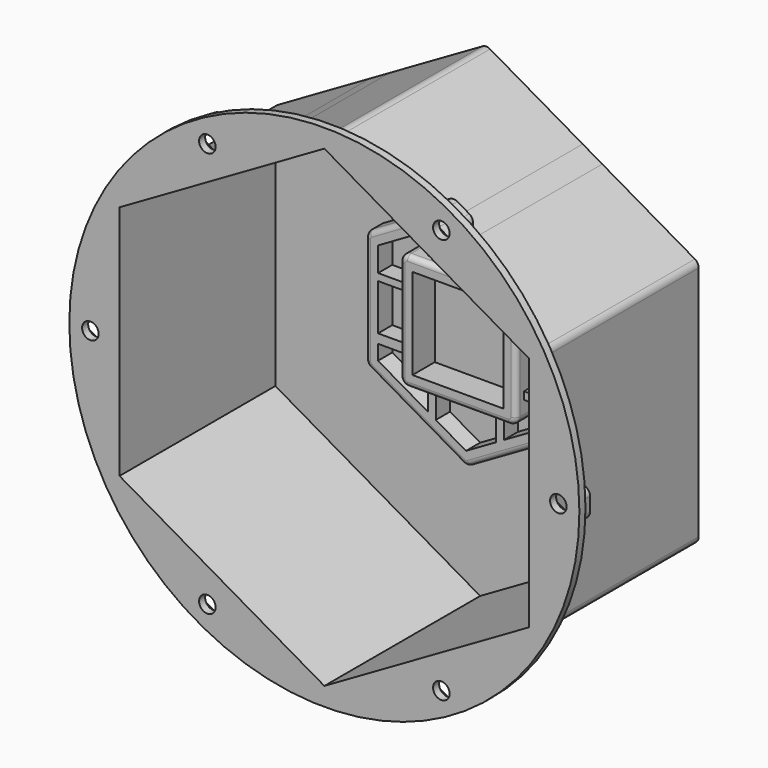
from build123d import *

# Parameters (mm, degrees)
F0_W      = 11.764
F0_H      = 3
F0_H_2    = 23.8
F0_H_3    = 3.6298790947
F0_H_4    = 18.1494033895
F0_H_5    = 2.7701719664
F1_DEPTH  = 3
F0_W_2    = 35.8
F0_H_6    = 35.8
F2_DEPTH  = 10
F3_DEPTH  = 79.8
F4_START  = 76.8
F0_R      = 100.55
F4_DEPTH  = 3
F5_R      = 2
F6_START  = 73.8
F0_W_3    = 0.8
F0_H_7    = 8.8911941455
F6_DEPTH  = 6
F7_D      = 6.5278
F8_DEPTH  = 14
F9_R      = 2
F10_DEPTH = 10


with BuildPart() as f1:
    # F0 (on Front) → F1 (new body)
    with BuildSketch(Plane.XZ):
        Polygon((0, -93.2420684741), (80.75, -46.6210342371), (80.75, 46.6210342371), (0, 93.2420684741), (-80.75, 46.6210342371), (-80.75, -46.6210342371), align=None)
        with BuildLine():
            ThreePointArc((39.664, -21.1679702696), (39.2620762114, -22.6679702696), (38.164, -23.7660464809))
            Line((38.164, -23.7660464809), (1.5, -44.9340167505))
            ThreePointArc((1.5, -44.9340167505), (0, -45.3359405391), (-1.5, -44.9340167505))
            Line((-1.5, -44.9340167505), (-38.164, -23.7660464809))
            ThreePointArc((-38.164, -23.7660464809), (-39.2620762114, -22.6679702696), (-39.664, -21.1679702696))
            Line((-39.664, -21.1679702696), (-39.664, 21.1679702696))
            ThreePointArc((-39.664, 21.1679702696), (-39.2620762114, 22.6679702696), (-38.164, 23.7660464809))
            Line((-38.164, 23.7660464809), (-1.5, 44.9340167505))
            ThreePointArc((-1.5, 44.9340167505), (0, 45.3359405391), (1.5, 44.9340167505))
            Line((1.5, 44.9340167505), (2.7712812921, 44.2000421543))
            Line((2.7712812921, 44.2000421543), (5.8889727457, 42.4000421543))
            Line((5.8889727457, 42.4000421543), (33.7750272543, 26.3000210771))
            Line((33.7750272543, 26.3000210771), (36.8927187079, 24.5000210771))
            Line((36.8927187079, 24.5000210771), (38.164, 23.7660464809))
            ThreePointArc((38.164, 23.7660464809), (39.2620762114, 22.6679702696), (39.664, 21.1679702696))
            Line((39.664, 21.1679702696), (39.664, -21.1679702696))
        make_face(mode=Mode.SUBTRACT)
        with BuildLine():
            Line((34.664, -20.0132697312), (34.664, -14.9))
            Line((34.664, -14.9), (22.9, -14.9))
            Line((22.9, -14.9), (22.9, -19.9))
            ThreePointArc((22.9, -19.9), (22.0213203436, -22.0213203436), (19.9, -22.9))
            Line((19.9, -22.9), (14.9, -22.9))
            Line((14.9, -22.9), (14.9, -31.4240204515))
            Line((14.9, -31.4240204515), (34.664, -20.0132697312))
        make_face()
        Polygon((11.9, -33.156071259), (14.9, -31.4240204515), (14.9, -22.9), (11.9, -22.9), align=None)
        Polygon((0, -40.0265394624), (11.9, -33.156071259), (11.9, -22.9), (-11.9, -22.9), (-11.9, -33.156071259), align=None)
        with BuildLine():
            Line((-14.9, 22.9), (-14.9, 31.4240204515))
            Line((-14.9, 31.4240204515), (-34.664, 20.0132697312))
            Line((-34.664, 20.0132697312), (-34.664, 10.4067251086))
            Line((-34.664, 10.4067251086), (-22.9, 10.4067251086))
            Line((-22.9, 10.4067251086), (-22.9, 19.9))
            ThreePointArc((-22.9, 19.9), (-22.0213203436, 22.0213203436), (-19.9, 22.9))
            Line((-19.9, 22.9), (-14.9, 22.9))
        make_face()
        Polygon((-11.9, 22.9), (-11.9, 33.156071259), (-14.9, 31.4240204515), (-14.9, 22.9), align=None)
        Polygon((11.9, 33.156071259), (3.3889727457, 38.0699151354), (0.2712812921, 39.8699151354), (0, 40.0265394624), (-11.9, 33.156071259), (-11.9, 22.9), (11.9, 22.9), align=None)
        Polygon((14.9, 22.9), (14.9, 31.4240204515), (11.9, 33.156071259), (11.9, 22.9), align=None)
        with BuildLine():
            Line((34.664, 20.0132697312), (34.3927187079, 20.1698940582))
            Line((34.3927187079, 20.1698940582), (31.2750272543, 21.9698940582))
            Line((31.2750272543, 21.9698940582), (14.9, 31.4240204515))
            Line((14.9, 31.4240204515), (14.9, 22.9))
            Line((14.9, 22.9), (19.9, 22.9))
            ThreePointArc((19.9, 22.9), (22.0213203436, 22.0213203436), (22.9, 19.9))
            Line((22.9, 19.9), (22.9, 14.9))
            Line((22.9, 14.9), (34.664, 14.9))
            Line((34.664, 14.9), (34.664, 20.0132697312))
        make_face()
        with Locations((28.782, 13.4)):
            Rectangle(F0_W, F0_H)
        with Locations((28.782, 0)):
            Rectangle(F0_W, F0_H_2)
        with Locations((28.782, -13.4)):
            Rectangle(F0_W, F0_H)
        Polygon((-14.9, -31.4240204515), (-11.9, -33.156071259), (-11.9, -22.9), (-14.9, -22.9), align=None)
        with BuildLine():
            Line((-22.9, -14.142729342), (-34.664, -14.142729342))
            Line((-34.664, -14.142729342), (-34.664, -20.0132697312))
            Line((-34.664, -20.0132697312), (-14.9, -31.4240204515))
            Line((-14.9, -31.4240204515), (-14.9, -22.9))
            Line((-14.9, -22.9), (-19.9, -22.9))
            ThreePointArc((-19.9, -22.9), (-22.0213203436, -22.0213203436), (-22.9, -19.9))
            Line((-22.9, -19.9), (-22.9, -14.142729342))
        make_face()
        with Locations((-28.782, -12.3277897947)):
            Rectangle(F0_W, F0_H_3)
        with Locations((-28.782, -1.4381485526)):
            Rectangle(F0_W, F0_H_4)
        with Locations((-28.782, 9.0216391254)):
            Rectangle(F0_W, F0_H_5)
        Polygon((3.3889727457, 38.0699151354), (5.8889727457, 42.4000421543), (2.7712812921, 44.2000421543), (0.2712812921, 39.8699151354), align=None)
        Polygon((34.3927187079, 20.1698940582), (36.8927187079, 24.5000210771), (33.7750272543, 26.3000210771), (31.2750272543, 21.9698940582), align=None)
    extrude(amount=F1_DEPTH)

    # F0 (on Front) → F2 (join)
    with BuildSketch(Plane.XZ):
        with BuildLine():
            Line((1.5, -44.9340167505), (38.164, -23.7660464809))
            ThreePointArc((38.164, -23.7660464809), (39.2620762114, -22.6679702696), (39.664, -21.1679702696))
            Line((39.664, -21.1679702696), (39.664, 21.1679702696))
            ThreePointArc((39.664, 21.1679702696), (39.2620762114, 22.6679702696), (38.164, 23.7660464809))
            Line((38.164, 23.7660464809), (36.8927187079, 24.5000210771))
            Line((36.8927187079, 24.5000210771), (34.3927187079, 20.1698940582))
            Line((34.3927187079, 20.1698940582), (34.664, 20.0132697312))
            Line((34.664, 20.0132697312), (34.664, 14.9))
            Line((34.664, 14.9), (34.664, 11.9))
            Line((34.664, 11.9), (34.664, -11.9))
            Line((34.664, -11.9), (34.664, -14.9))
            Line((34.664, -14.9), (34.664, -20.0132697312))
            Line((34.664, -20.0132697312), (14.9, -31.4240204515))
            Line((14.9, -31.4240204515), (11.9, -33.156071259))
            Line((11.9, -33.156071259), (0, -40.0265394624))
            Line((0, -40.0265394624), (-11.9, -33.156071259))
            Line((-11.9, -33.156071259), (-14.9, -31.4240204515))
            Line((-14.9, -31.4240204515), (-34.664, -20.0132697312))
            Line((-34.664, -20.0132697312), (-34.664, -14.142729342))
            Line((-34.664, -14.142729342), (-34.664, -10.5128502473))
            Line((-34.664, -10.5128502473), (-34.664, 7.6365531422))
            Line((-34.664, 7.6365531422), (-34.664, 10.4067251086))
            Line((-34.664, 10.4067251086), (-34.664, 20.0132697312))
            Line((-34.664, 20.0132697312), (-14.9, 31.4240204515))
            Line((-14.9, 31.4240204515), (-11.9, 33.156071259))
            Line((-11.9, 33.156071259), (0, 40.0265394624))
            Line((0, 40.0265394624), (0.2712812921, 39.8699151354))
            Line((0.2712812921, 39.8699151354), (2.7712812921, 44.2000421543))
            Line((2.7712812921, 44.2000421543), (1.5, 44.9340167505))
            ThreePointArc((1.5, 44.9340167505), (0, 45.3359405391), (-1.5, 44.9340167505))
            Line((-1.5, 44.9340167505), (-38.164, 23.7660464809))
            ThreePointArc((-38.164, 23.7660464809), (-39.2620762114, 22.6679702696), (-39.664, 21.1679702696))
            Line((-39.664, 21.1679702696), (-39.664, -21.1679702696))
            ThreePointArc((-39.664, -21.1679702696), (-39.2620762114, -22.6679702696), (-38.164, -23.7660464809))
            Line((-38.164, -23.7660464809), (-1.5, -44.9340167505))
            ThreePointArc((-1.5, -44.9340167505), (0, -45.3359405391), (1.5, -44.9340167505))
        make_face()
    extrude(amount=F2_DEPTH)

    # F0 (on Front) → F3 (join)
    with BuildSketch(Plane.XZ):
        with BuildLine():
            Line((83.75, 4.4455970728), (83.75, 46.6210342371))
            ThreePointArc((83.75, 46.6210342371), (83.3480762114, 48.1210342371), (82.25, 49.2191104484))
            Line((82.25, 49.2191104484), (45.725, 70.3068290306))
            Line((45.725, 70.3068290306), (38.025, 74.7524261033))
            Line((38.025, 74.7524261033), (1.5, 95.8401446855))
            ThreePointArc((1.5, 95.8401446855), (0, 96.2420684741), (-1.5, 95.8401446855))
            Line((-1.5, 95.8401446855), (-38.025, 74.7524261033))
            Line((-38.025, 74.7524261033), (-45.725, 70.3068290306))
            Line((-45.725, 70.3068290306), (-82.25, 49.2191104484))
            ThreePointArc((-82.25, 49.2191104484), (-83.3480762114, 48.1210342371), (-83.75, 46.6210342371))
            Line((-83.75, 46.6210342371), (-83.75, 4.1800841187))
            Line((-83.75, 4.1800841187), (-83.75, -3.9581455377))
            Line((-83.75, -3.9581455377), (-83.75, -46.6210342371))
            ThreePointArc((-83.75, -46.6210342371), (-83.3480762114, -48.1210342371), (-82.25, -49.2191104484))
            Line((-82.25, -49.2191104484), (-45.7833874392, -70.2731190268))
            Line((-45.7833874392, -70.2731190268), (-38.0831462279, -74.718855363))
            Line((-38.0831462279, -74.718855363), (-1.5, -95.8401446855))
            ThreePointArc((-1.5, -95.8401446855), (0, -96.2420684741), (1.5, -95.8401446855))
            Line((1.5, -95.8401446855), (38.1444882108, -74.6834395526))
            Line((38.1444882108, -74.6834395526), (45.8568599601, -70.2306996471))
            Line((45.8568599601, -70.2306996471), (82.25, -49.2191104484))
            ThreePointArc((82.25, -49.2191104484), (83.3480762114, -48.1210342371), (83.75, -46.6210342371))
            Line((83.75, -46.6210342371), (83.75, -4.4455970728))
            Line((83.75, -4.4455970728), (83.75, 4.4455970728))
        make_face()
        Polygon((80.75, 46.6210342371), (80.75, -46.6210342371), (0, -93.2420684741), (-80.75, -46.6210342371), (-80.75, 46.6210342371), (0, 93.2420684741), align=None, mode=Mode.SUBTRACT)
    extrude(amount=F3_DEPTH)

    # F0 (on Front) → F4 (join)
    with BuildSketch(Plane.XZ.offset(F4_START)):
        Circle(F0_R)
        with BuildLine():
            ThreePointArc((82.25, 49.2191104484), (83.3480762114, 48.1210342371), (83.75, 46.6210342371))
            Line((83.75, 46.6210342371), (83.75, 4.4455970728))
            Line((83.75, 4.4455970728), (84.55, 4.4455970728))
            Line((84.55, 4.4455970728), (90.75, 8.0251687417))
            ThreePointArc((90.75, 8.0251687417), (92.25, 8.4270925304), (93.75, 8.0251687417))
            Line((93.75, 8.0251687417), (98.45, 5.3116224765))
            ThreePointArc((98.45, 5.3116224765), (99.5480762114, 4.2135462652), (99.95, 2.7135462652))
            Line((99.95, 2.7135462652), (99.95, -2.7135462652))
            ThreePointArc((99.95, -2.7135462652), (99.5480762114, -4.2135462652), (98.45, -5.3116224765))
            Line((98.45, -5.3116224765), (93.75, -8.0251687417))
            ThreePointArc((93.75, -8.0251687417), (92.25, -8.4270925304), (90.75, -8.0251687417))
            Line((90.75, -8.0251687417), (84.55, -4.4455970728))
            Line((84.55, -4.4455970728), (83.75, -4.4455970728))
            Line((83.75, -4.4455970728), (83.75, -46.6210342371))
            ThreePointArc((83.75, -46.6210342371), (83.3480762114, -48.1210342371), (82.25, -49.2191104484))
            Line((82.25, -49.2191104484), (45.8568599601, -70.2306996471))
            Line((45.8568599601, -70.2306996471), (46.2835018729, -71.0010622594))
            Line((46.2835018729, -71.0010622594), (52.4187041842, -74.6905914884))
            ThreePointArc((52.4187041842, -74.6905914884), (53.4970306734, -75.8080684299), (53.8721503359, -77.3149950939))
            Line((53.8721503359, -77.3149950939), (53.7754024395, -82.7412252012))
            ThreePointArc((53.7754024395, -82.7412252012), (53.3468022646, -84.2338218051), (52.2293253232, -85.3121482943))
            Line((52.2293253232, -85.3121482943), (47.4816982552, -87.9414772119))
            ThreePointArc((47.4816982552, -87.9414772119), (45.9747715912, -88.3165968744), (44.4821749873, -87.8879966995))
            Line((44.4821749873, -87.8879966995), (39.8312958158, -85.0910955098))
            ThreePointArc((39.8312958158, -85.0910955098), (38.7529693266, -83.9736185684), (38.3778496641, -82.4666919043))
            Line((38.3778496641, -82.4666919043), (38.5054745488, -75.3086862308))
            Line((38.5054745488, -75.3086862308), (38.1444882108, -74.6834395526))
            Line((38.1444882108, -74.6834395526), (1.5, -95.8401446855))
            ThreePointArc((1.5, -95.8401446855), (0, -96.2420684741), (-1.5, -95.8401446855))
            Line((-1.5, -95.8401446855), (-38.0831462279, -74.718855363))
            Line((-38.0831462279, -74.718855363), (-38.460428699, -75.3844391559))
            Line((-38.460428699, -75.3844391559), (-38.4037631222, -82.5433582325))
            ThreePointArc((-38.4037631222, -82.5433582325), (-38.79380162, -84.0464925253), (-39.8831520139, -85.1532257593))
            Line((-39.8831520139, -85.1532257593), (-44.5615267041, -87.9038881506))
            ThreePointArc((-44.5615267041, -87.9038881506), (-46.0582984359, -88.3176720495), (-47.5614327287, -87.9276335517))
            Line((-47.5614327287, -87.9276335517), (-52.2827635819, -85.2513734172))
            ThreePointArc((-52.2827635819, -85.2513734172), (-53.3894968159, -84.1620230233), (-53.8032807148, -82.6652512916))
            Line((-53.8032807148, -82.6652512916), (-53.8462368778, -77.2383287657))
            ThreePointArc((-53.8462368778, -77.2383287657), (-53.45619838, -75.7351944729), (-52.3668479861, -74.628461239))
            Line((-52.3668479861, -74.628461239), (-46.1953749905, -70.9999278717))
            Line((-46.1953749905, -70.9999278717), (-45.7833874392, -70.2731190268))
            Line((-45.7833874392, -70.2731190268), (-82.25, -49.2191104484))
            ThreePointArc((-82.25, -49.2191104484), (-83.3480762114, -48.1210342371), (-83.75, -46.6210342371))
            Line((-83.75, -46.6210342371), (-83.75, -3.9581455377))
            Line((-83.75, -3.9581455377), (-85.1501733085, -3.9764250951))
            Line((-85.1501733085, -3.9764250951), (-90.6552047962, -7.2513100663))
            ThreePointArc((-90.6552047962, -7.2513100663), (-92.149830231, -7.6727807551), (-93.654949171, -7.290472361))
            Line((-93.654949171, -7.290472361), (-97.7324211262, -5.0067881935))
            ThreePointArc((-97.7324211262, -5.0067881935), (-98.844738167, -3.9231399422), (-99.2662088558, -2.4285145074))
            Line((-99.2662088558, -2.4285145074), (-99.3272163301, 2.2445218728))
            ThreePointArc((-99.3272163301, 2.2445218728), (-98.9449079361, 3.7496408129), (-97.8612596847, 4.8619578537))
            Line((-97.8612596847, 4.8619578537), (-93.8447952038, 7.2513100663))
            ThreePointArc((-93.8447952038, 7.2513100663), (-92.350169769, 7.6727807551), (-90.845050829, 7.290472361))
            Line((-90.845050829, 7.290472361), (-85.2564015056, 4.1604177297))
            Line((-85.2564015056, 4.1604177297), (-83.75, 4.1800841187))
            Line((-83.75, 4.1800841187), (-83.75, 46.6210342371))
            ThreePointArc((-83.75, 46.6210342371), (-83.3480762114, 48.1210342371), (-82.25, 49.2191104484))
            Line((-82.25, 49.2191104484), (-45.725, 70.3068290306))
            Line((-45.725, 70.3068290306), (-46.125, 70.9996493536))
            Line((-46.125, 70.9996493536), (-52.325, 74.5792210226))
            ThreePointArc((-52.325, 74.5792210226), (-53.4230762114, 75.6772972339), (-53.825, 77.1772972339))
            Line((-53.825, 77.1772972339), (-53.825, 82.6043897643))
            ThreePointArc((-53.825, 82.6043897643), (-53.4230762114, 84.1043897643), (-52.325, 85.2024659757))
            Line((-52.325, 85.2024659757), (-47.625, 87.9160122409))
            ThreePointArc((-47.625, 87.9160122409), (-46.125, 88.3179360295), (-44.625, 87.9160122409))
            Line((-44.625, 87.9160122409), (-39.925, 85.2024659757))
            ThreePointArc((-39.925, 85.2024659757), (-38.8269237886, 84.1043897643), (-38.425, 82.6043897643))
            Line((-38.425, 82.6043897643), (-38.425, 75.4452464264))
            Line((-38.425, 75.4452464264), (-38.025, 74.7524261033))
            Line((-38.025, 74.7524261033), (-1.5, 95.8401446855))
            ThreePointArc((-1.5, 95.8401446855), (0, 96.2420684741), (1.5, 95.8401446855))
            Line((1.5, 95.8401446855), (38.025, 74.7524261033))
            Line((38.025, 74.7524261033), (38.425, 75.4452464264))
            Line((38.425, 75.4452464264), (38.425, 82.6043897643))
            ThreePointArc((38.425, 82.6043897643), (38.8269237886, 84.1043897643), (39.925, 85.2024659757))
            Line((39.925, 85.2024659757), (44.625, 87.9160122409))
            ThreePointArc((44.625, 87.9160122409), (46.125, 88.3179360295), (47.625, 87.9160122409))
            Line((47.625, 87.9160122409), (52.325, 85.2024659757))
            ThreePointArc((52.325, 85.2024659757), (53.4230762114, 84.1043897643), (53.825, 82.6043897643))
            Line((53.825, 82.6043897643), (53.825, 77.1772972339))
            ThreePointArc((53.825, 77.1772972339), (53.4230762114, 75.6772972339), (52.325, 74.5792210226))
            Line((52.325, 74.5792210226), (46.125, 70.9996493536))
            Line((46.125, 70.9996493536), (45.725, 70.3068290306))
            Line((45.725, 70.3068290306), (82.25, 49.2191104484))
        make_face(mode=Mode.SUBTRACT)
    extrude(amount=F4_DEPTH)

    # F5
    f5_edges = [f1.edges().sort_by_distance(p)[0] for p in [
        (2.135641, -10, 44.567029),
        (37.528359, -10, 24.133034),
    ]]
    fillet(f5_edges, radius=F5_R)



with BuildPart() as f1b:
    # F0 (on Front) → F1, piece 2 (new body)
    with BuildSketch(Plane.XZ):
        Rectangle(F0_W_2, F0_H_6)
    extrude(amount=F1_DEPTH)


with BuildPart() as f4:
    # F0 (on Front) → F4, piece 2 (new body)
    with BuildSketch(Plane.XZ.offset(F4_START)):
        Polygon((-46.2600288495, 73.3104356691), (-40.4937140766, 76.4837011702), (-40.3586852272, 83.0641090003), (-45.9899711505, 86.4712513292), (-51.7562859234, 83.297985828), (-51.8913147728, 76.717577998), align=None)
    extrude(amount=F4_DEPTH)


with BuildPart() as f4b:
    # F0 (on Front) → F4, piece 3 (new body)
    with BuildSketch(Plane.XZ.offset(F4_START)):
        Polygon((51.825, 76.5999469647), (51.825, 83.1817400335), (46.125, 86.4726365679), (40.425, 83.1817400335), (40.425, 76.5999469647), (46.125, 73.3090504304), align=None)
    extrude(amount=F4_DEPTH)


with BuildPart() as f4c:
    # F0 (on Front) → F4, piece 4 (new body)
    with BuildSketch(Plane.XZ.offset(F4_START)):
        Polygon((92.25, -6.5817930688), (97.95, -3.2908965344), (97.95, 3.2908965344), (92.25, 6.5817930688), (86.55, 3.2908965344), (86.55, -3.2908965344), align=None)
    extrude(amount=F4_DEPTH)


with BuildPart() as f4d:
    # F0 (on Front) → F4, piece 5 (new body)
    with BuildSketch(Plane.XZ.offset(F4_START)):
        Polygon((46.0076674448, -86.4715906506), (51.7654279314, -83.2828300484), (51.8827604867, -76.7020828969), (46.2423325552, -73.3100963477), (40.4845720686, -76.4988569499), (40.3672395133, -83.0796041013), align=None)
    extrude(amount=F4_DEPTH)


with BuildPart() as f4e:
    # F0 (on Front) → F4, piece 6 (new body)
    with BuildSketch(Plane.XZ.offset(F4_START)):
        Polygon((-46.0729042278, -86.4724303921), (-40.3991306673, -83.1365206835), (-40.4512264395, -76.5549337905), (-46.1770957722, -73.3092566061), (-51.8508693327, -76.6451663147), (-51.7987735605, -83.2267532078), align=None)
    extrude(amount=F4_DEPTH)


with BuildPart() as f4f:
    # F0 (on Front) → F4, piece 7 (new body)
    with BuildSketch(Plane.XZ.offset(F4_START)):
        Polygon((-92.1640806267, -6.5812322449), (-86.5075260011, -3.2162077625), (-86.5934453744, 3.3650244824), (-92.3359193733, 6.5812322449), (-97.9924739989, 3.2162077625), (-97.9065546256, -3.3650244824), align=None)
    extrude(amount=F4_DEPTH)


with BuildPart() as f1_1:
    add(f1.part)

    add(f4.part)  # F6 merges F4

    add(f4b.part)  # F6 merges F4b

    add(f4c.part)  # F6 merges F4c

    add(f4d.part)  # F6 merges F4d

    add(f4e.part)  # F6 merges F4e

    add(f4f.part)  # F6 merges F4f
    # F0 (on Front) → F6 (join)
    with BuildSketch(Plane.XZ.offset(F6_START)):
        with BuildLine():
            Line((-46.125, 70.9996493536), (-38.425, 75.4452464264))
            Line((-38.425, 75.4452464264), (-38.425, 82.6043897643))
            ThreePointArc((-38.425, 82.6043897643), (-38.8269237886, 84.1043897643), (-39.925, 85.2024659757))
            Line((-39.925, 85.2024659757), (-44.625, 87.9160122409))
            ThreePointArc((-44.625, 87.9160122409), (-46.125, 88.3179360295), (-47.625, 87.9160122409))
            Line((-47.625, 87.9160122409), (-52.325, 85.2024659757))
            ThreePointArc((-52.325, 85.2024659757), (-53.4230762114, 84.1043897643), (-53.825, 82.6043897643))
            Line((-53.825, 82.6043897643), (-53.825, 77.1772972339))
            ThreePointArc((-53.825, 77.1772972339), (-53.4230762114, 75.6772972339), (-52.325, 74.5792210226))
            Line((-52.325, 74.5792210226), (-46.125, 70.9996493536))
        make_face()
        Polygon((-40.3586852272, 83.0641090003), (-40.4937140766, 76.4837011702), (-46.2600288495, 73.3104356691), (-51.8913147728, 76.717577998), (-51.7562859234, 83.297985828), (-45.9899711505, 86.4712513292), align=None, mode=Mode.SUBTRACT)
        Polygon((-45.725, 70.3068290306), (-38.025, 74.7524261033), (-38.425, 75.4452464264), (-46.125, 70.9996493536), align=None)
        with BuildLine():
            Line((38.425, 75.4452464264), (46.125, 70.9996493536))
            Line((46.125, 70.9996493536), (52.325, 74.5792210226))
            ThreePointArc((52.325, 74.5792210226), (53.4230762114, 75.6772972339), (53.825, 77.1772972339))
            Line((53.825, 77.1772972339), (53.825, 82.6043897643))
            ThreePointArc((53.825, 82.6043897643), (53.4230762114, 84.1043897643), (52.325, 85.2024659757))
            Line((52.325, 85.2024659757), (47.625, 87.9160122409))
            ThreePointArc((47.625, 87.9160122409), (46.125, 88.3179360295), (44.625, 87.9160122409))
            Line((44.625, 87.9160122409), (39.925, 85.2024659757))
            ThreePointArc((39.925, 85.2024659757), (38.8269237886, 84.1043897643), (38.425, 82.6043897643))
            Line((38.425, 82.6043897643), (38.425, 75.4452464264))
        make_face()
        Polygon((46.125, 86.4726365679), (51.825, 83.1817400335), (51.825, 76.5999469647), (46.125, 73.3090504304), (40.425, 76.5999469647), (40.425, 83.1817400335), align=None, mode=Mode.SUBTRACT)
        Polygon((38.025, 74.7524261033), (45.725, 70.3068290306), (46.125, 70.9996493536), (38.425, 75.4452464264), align=None)
        with BuildLine():
            Line((90.75, 8.0251687417), (84.55, 4.4455970728))
            Line((84.55, 4.4455970728), (84.55, -4.4455970728))
            Line((84.55, -4.4455970728), (90.75, -8.0251687417))
            ThreePointArc((90.75, -8.0251687417), (92.25, -8.4270925304), (93.75, -8.0251687417))
            Line((93.75, -8.0251687417), (98.45, -5.3116224765))
            ThreePointArc((98.45, -5.3116224765), (99.5480762114, -4.2135462652), (99.95, -2.7135462652))
            Line((99.95, -2.7135462652), (99.95, 2.7135462652))
            ThreePointArc((99.95, 2.7135462652), (99.5480762114, 4.2135462652), (98.45, 5.3116224765))
            Line((98.45, 5.3116224765), (93.75, 8.0251687417))
            ThreePointArc((93.75, 8.0251687417), (92.25, 8.4270925304), (90.75, 8.0251687417))
        make_face()
        Polygon((97.95, 3.2908965344), (97.95, -3.2908965344), (92.25, -6.5817930688), (86.55, -3.2908965344), (86.55, 3.2908965344), (92.25, 6.5817930688), align=None, mode=Mode.SUBTRACT)
        with Locations((84.15, 0)):
            Rectangle(F0_W_3, F0_H_7)
        with BuildLine():
            Line((52.4187041842, -74.6905914884), (46.2835018729, -71.0010622594))
            Line((46.2835018729, -71.0010622594), (38.5054745488, -75.3086862308))
            Line((38.5054745488, -75.3086862308), (38.3778496641, -82.4666919043))
            ThreePointArc((38.3778496641, -82.4666919043), (38.7529693266, -83.9736185684), (39.8312958158, -85.0910955098))
            Line((39.8312958158, -85.0910955098), (44.4821749873, -87.8879966995))
            ThreePointArc((44.4821749873, -87.8879966995), (45.9747715912, -88.3165968744), (47.4816982552, -87.9414772119))
            Line((47.4816982552, -87.9414772119), (52.2293253232, -85.3121482943))
            ThreePointArc((52.2293253232, -85.3121482943), (53.3468022646, -84.2338218051), (53.7754024395, -82.7412252012))
            Line((53.7754024395, -82.7412252012), (53.8721503359, -77.3149950939))
            ThreePointArc((53.8721503359, -77.3149950939), (53.4970306734, -75.8080684299), (52.4187041842, -74.6905914884))
        make_face()
        Polygon((51.8827604867, -76.7020828969), (51.7654279314, -83.2828300484), (46.0076674448, -86.4715906506), (40.3672395133, -83.0796041013), (40.4845720686, -76.4988569499), (46.2423325552, -73.3100963477), align=None, mode=Mode.SUBTRACT)
        Polygon((46.2835018729, -71.0010622594), (45.8568599601, -70.2306996471), (38.1444882108, -74.6834395526), (38.5054745488, -75.3086862308), align=None)
        with BuildLine():
            Line((-38.4037631222, -82.5433582325), (-38.460428699, -75.3844391559))
            Line((-38.460428699, -75.3844391559), (-46.1953749905, -70.9999278717))
            Line((-46.1953749905, -70.9999278717), (-52.3668479861, -74.628461239))
            ThreePointArc((-52.3668479861, -74.628461239), (-53.45619838, -75.7351944729), (-53.8462368778, -77.2383287657))
            Line((-53.8462368778, -77.2383287657), (-53.8032807148, -82.6652512916))
            ThreePointArc((-53.8032807148, -82.6652512916), (-53.3894968159, -84.1620230233), (-52.2827635819, -85.2513734172))
            Line((-52.2827635819, -85.2513734172), (-47.5614327287, -87.9276335517))
            ThreePointArc((-47.5614327287, -87.9276335517), (-46.0582984359, -88.3176720495), (-44.5615267041, -87.9038881506))
            Line((-44.5615267041, -87.9038881506), (-39.8831520139, -85.1532257593))
            ThreePointArc((-39.8831520139, -85.1532257593), (-38.79380162, -84.0464925253), (-38.4037631222, -82.5433582325))
        make_face()
        Polygon((-40.4512264395, -76.5549337905), (-40.3991306673, -83.1365206835), (-46.0729042278, -86.4724303921), (-51.7987735605, -83.2267532078), (-51.8508693327, -76.6451663147), (-46.1770957722, -73.3092566061), align=None, mode=Mode.SUBTRACT)
        Polygon((-38.460428699, -75.3844391559), (-38.0831462279, -74.718855363), (-45.7833874392, -70.2731190268), (-46.1953749905, -70.9999278717), align=None)
        with BuildLine():
            Line((-85.1501733085, -3.9764250951), (-85.2564015056, 4.1604177297))
            Line((-85.2564015056, 4.1604177297), (-90.845050829, 7.290472361))
            ThreePointArc((-90.845050829, 7.290472361), (-92.350169769, 7.6727807551), (-93.8447952038, 7.2513100663))
            Line((-93.8447952038, 7.2513100663), (-97.8612596847, 4.8619578537))
            ThreePointArc((-97.8612596847, 4.8619578537), (-98.9449079361, 3.7496408129), (-99.3272163301, 2.2445218728))
            Line((-99.3272163301, 2.2445218728), (-99.2662088558, -2.4285145074))
            ThreePointArc((-99.2662088558, -2.4285145074), (-98.844738167, -3.9231399422), (-97.7324211262, -5.0067881935))
            Line((-97.7324211262, -5.0067881935), (-93.654949171, -7.290472361))
            ThreePointArc((-93.654949171, -7.290472361), (-92.149830231, -7.6727807551), (-90.6552047962, -7.2513100663))
            Line((-90.6552047962, -7.2513100663), (-85.1501733085, -3.9764250951))
        make_face()
        Polygon((-86.5934453744, 3.3650244824), (-86.5075260011, -3.2162077625), (-92.1640806267, -6.5812322449), (-97.9065546256, -3.3650244824), (-97.9924739989, 3.2162077625), (-92.3359193733, 6.5812322449), align=None, mode=Mode.SUBTRACT)
        Polygon((-83.75, -3.9581455377), (-83.75, 4.1800841187), (-85.2564015056, 4.1604177297), (-85.1501733085, -3.9764250951), align=None)
    extrude(amount=F6_DEPTH)

    # F7 (through all)
    with Locations(Plane(origin=(0, 0, 0), x_dir=(1, 0, 0), z_dir=(0, 1, 0))):
        with Locations((-46.125, -79.8908434991), (46.125, -79.8908434991), (92.25, 0), (46.125, 79.8908434991), (-46.125, 79.8908434991), (-92.25, 0)):
            Hole(F7_D / 2)


    add(f1b.part)  # F8 merges F1b
    # F0 (on Front) → F8 (join)
    with BuildSketch(Plane.XZ):
        with BuildLine():
            Line((19.9, 22.9), (14.9, 22.9))
            Line((14.9, 22.9), (11.9, 22.9))
            Line((11.9, 22.9), (-11.9, 22.9))
            Line((-11.9, 22.9), (-14.9, 22.9))
            Line((-14.9, 22.9), (-19.9, 22.9))
            ThreePointArc((-19.9, 22.9), (-22.0213203436, 22.0213203436), (-22.9, 19.9))
            Line((-22.9, 19.9), (-22.9, 10.4067251086))
            Line((-22.9, 10.4067251086), (-22.9, 7.6365531422))
            Line((-22.9, 7.6365531422), (-22.9, -10.5128502473))
            Line((-22.9, -10.5128502473), (-22.9, -14.142729342))
            Line((-22.9, -14.142729342), (-22.9, -19.9))
            ThreePointArc((-22.9, -19.9), (-22.0213203436, -22.0213203436), (-19.9, -22.9))
            Line((-19.9, -22.9), (-14.9, -22.9))
            Line((-14.9, -22.9), (-11.9, -22.9))
            Line((-11.9, -22.9), (11.9, -22.9))
            Line((11.9, -22.9), (14.9, -22.9))
            Line((14.9, -22.9), (19.9, -22.9))
            ThreePointArc((19.9, -22.9), (22.0213203436, -22.0213203436), (22.9, -19.9))
            Line((22.9, -19.9), (22.9, -14.9))
            Line((22.9, -14.9), (22.9, -11.9))
            Line((22.9, -11.9), (22.9, 11.9))
            Line((22.9, 11.9), (22.9, 14.9))
            Line((22.9, 14.9), (22.9, 19.9))
            ThreePointArc((22.9, 19.9), (22.0213203436, 22.0213203436), (19.9, 22.9))
        make_face()
        Rectangle(F0_W_2, F0_H_6, mode=Mode.SUBTRACT)
    extrude(amount=F8_DEPTH)

    # F9
    f9_edges = [f1_1.edges().sort_by_distance(p)[0] for p in [
        (22.9, -14, 0),
        (-22.9, -14, 0),
        (-22.02132, -14, 22.02132),
        (0, -14, 22.9),
        (22.02132, -14, 22.02132),
        (22.02132, -14, -22.02132),
        (0, -14, -22.9),
        (-22.02132, -14, -22.02132),
    ]]
    fillet(f9_edges, radius=F9_R)

    # F0 (on Front) → F10 (join)
    with BuildSketch(Plane.XZ):
        with Locations((-28.782, -12.3277897947)):
            Rectangle(F0_W, F0_H_3)
        with Locations((-28.782, 9.0216391254)):
            Rectangle(F0_W, F0_H_5)
        Polygon((-11.9, 22.9), (-11.9, 33.156071259), (-14.9, 31.4240204515), (-14.9, 22.9), align=None)
        Polygon((14.9, 22.9), (14.9, 31.4240204515), (11.9, 33.156071259), (11.9, 22.9), align=None)
        with Locations((28.782, 13.4)):
            Rectangle(F0_W, F0_H)
        with Locations((28.782, -13.4)):
            Rectangle(F0_W, F0_H)
        Polygon((11.9, -33.156071259), (14.9, -31.4240204515), (14.9, -22.9), (11.9, -22.9), align=None)
        Polygon((-14.9, -31.4240204515), (-11.9, -33.156071259), (-11.9, -22.9), (-14.9, -22.9), align=None)
        Polygon((31.2750272543, 21.9698940582), (33.7750272543, 26.3000210771), (5.8889727457, 42.4000421543), (3.3889727457, 38.0699151354), (11.9, 33.156071259), (14.9, 31.4240204515), align=None)
    extrude(amount=F10_DEPTH)


solid = f1_1.part
